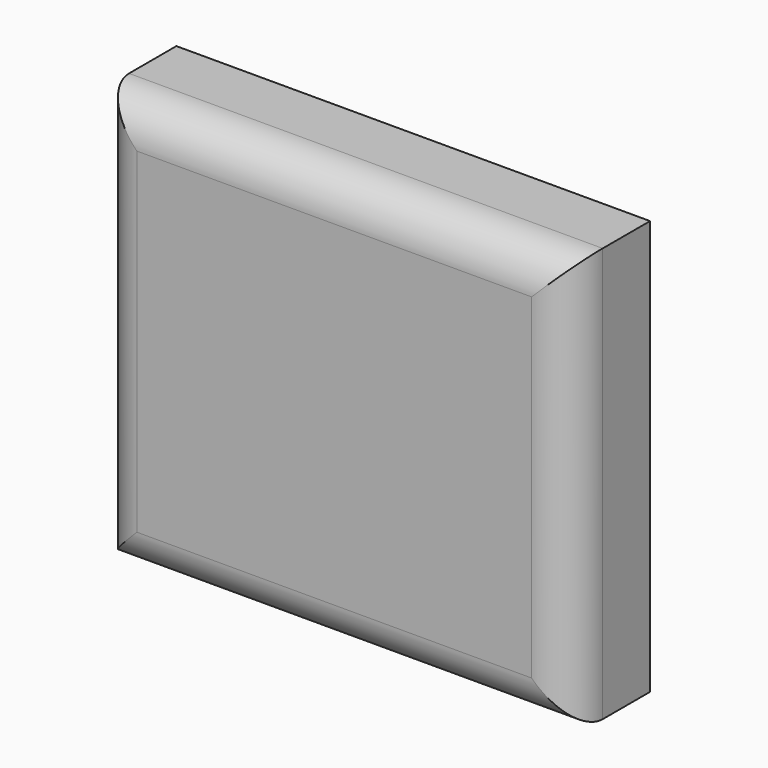
from build123d import *

# Parameters (mm, degrees)
F0_W     = 24
F0_H     = 21
F1_DEPTH = 5
F2_R     = 2


# Not quite as in the source:
# - a feature of the source that left no trace in its solid (it failed there, or was rolled back) is left out


with BuildPart() as f1:
    # F0 (on Front) → F1 (new body)
    with BuildSketch(Plane.XZ):
        with Locations((-12, 10.5)):
            Rectangle(F0_W, F0_H)
    extrude(amount=F1_DEPTH)

    # F2
    f2_edges = [f1.edges().sort_by_distance(p)[0] for p in [
        (-12, -5, 0),
        (0, -5, 10.5),
        (-12, -5, 21),
        (-24, -5, 10.5),
    ]]
    fillet(f2_edges, radius=F2_R)


solid = f1.part
